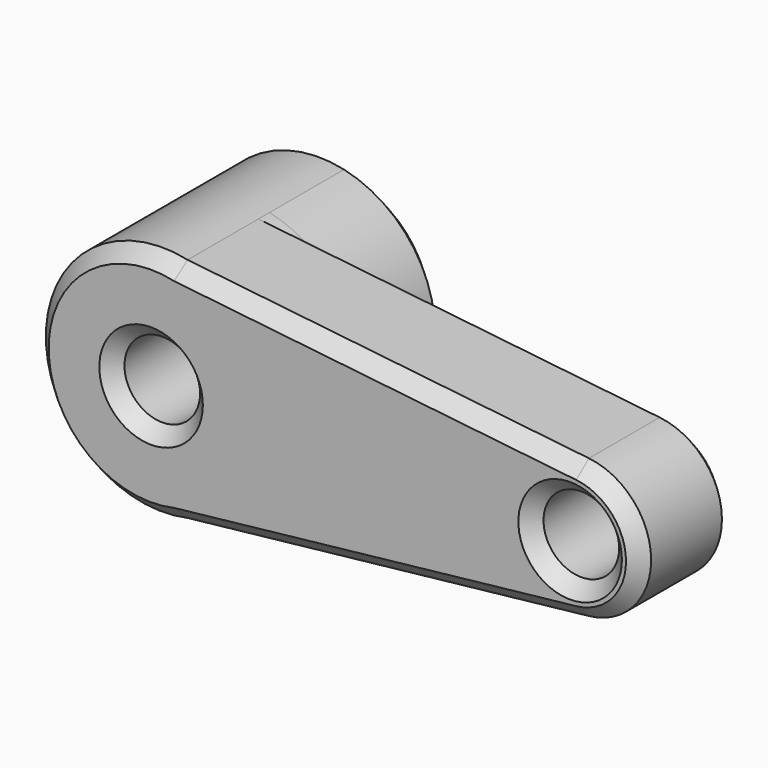
from build123d import *
from build123d import SkipClean  # not in build123d's __all__

# Parameters (mm, degrees)
F0_R         = 8.117177454
F1_DEPTH     = 25
F2_SIZE      = 3
F3_DEPTH     = 25
F4_SIZE      = 5
F5_T4_DEPTH  = 109.868464735
F5_S5_R      = 25
F5_T6_DEPTH  = 57
F5_T8_ANGLE  = 167.4336377222
F5_T12_DEPTH = 109.868464735
F5_S13_R     = 25
F5_T14_DEPTH = 57


# Not quite as in the source:
# - a fillet or chamfer that OpenCascade refuses, or shapes differently, is made with other operations: its cross-section is extruded or revolved along the edge and cut away or added


with BuildPart() as f1:
    # F0 (on Front) → F1 (new body)
    with BuildSketch(Plane.XZ):
        with BuildLine():
            ThreePointArc((5.4392563458, -24.4011165811), (19.5061709293, -15.6367930113), (25, 0))
            ThreePointArc((25, 0), (19.5061709293, 15.6367930113), (5.4392563458, 24.4011165811))
            ThreePointArc((5.4392563458, 24.4011165811), (-25, 0), (5.4392563458, -24.4011165811))
        make_face()
        Circle(F0_R, mode=Mode.SUBTRACT)
        with BuildLine():
            ThreePointArc((5.4392563458, 24.4011165811), (19.5061709293, 15.6367930113), (25, 0))
            ThreePointArc((25, 0), (19.5061709293, -15.6367930113), (5.4392563458, -24.4011165811))
            Line((5.4392563458, -24.4011165811), (91.6416380189, -14.909896868))
            ThreePointArc((91.6416380189, -14.909896868), (75, 0), (91.6416380189, 14.909896868))
            Line((91.6416380189, 14.909896868), (5.4392563458, 24.4011165811))
        make_face()
        with BuildLine():
            ThreePointArc((105, 0), (101.1719418698, 10.0093813424), (91.6416380189, 14.909896868))
            ThreePointArc((91.6416380189, 14.909896868), (75, 0), (91.6416380189, -14.909896868))
            ThreePointArc((91.6416380189, -14.909896868), (101.1719418698, -10.0093813424), (105, 0))
        make_face()
        with Locations((90, 0)):
            Circle(F0_R, mode=Mode.SUBTRACT)
    extrude(amount=F1_DEPTH)

    # F2
    f2_edges = [f1.edges().sort_by_distance(p)[0] for p in [
        (-25, -25, 0),
        (48.540447, -25, -19.655507),
        (105, -25, 0),
        (48.540447, -25, 19.655507),
        (-8.117177, -25, 0),
        (81.882823, -25, 0),
    ]]
    chamfer(f2_edges, length=F2_SIZE)

    # F0 (on Front) → F3 (join)
    with BuildSketch(Plane.XZ):
        with BuildLine():
            ThreePointArc((5.4392563458, -24.4011165811), (19.5061709293, -15.6367930113), (25, 0))
            ThreePointArc((25, 0), (19.5061709293, 15.6367930113), (5.4392563458, 24.4011165811))
            ThreePointArc((5.4392563458, 24.4011165811), (-25, 0), (5.4392563458, -24.4011165811))
        make_face()
        Circle(F0_R, mode=Mode.SUBTRACT)
    with SkipClean():  # cleaning this boolean's faces spoils the solid; the shape is the same uncleaned
        extrude(amount=-F3_DEPTH)

    # F4
    f4_edges = [f1.edges().sort_by_distance(p)[0] for p in [
        (-5.439256, 25, 24.401117),
        (-8.117177, 25, 0),
    ]]
    chamfer(f4_edges, length=F4_SIZE)

    # F5: chamfer of 3 on 1 edges, made by hand


with BuildPart() as f5_tool2:
    # F5_s3 → F5_t4 (new body)
    with BuildSketch(Plane(origin=(88.922009846, 0, -9.7906614225), x_dir=(0, 1, 0), z_dir=(-0.9939931245, 0, 0.1094425346))):
        Polygon((0, -21.8498281134), (-3, -24.8498281134), (0, -24.8498281134), align=None)
    extrude(amount=F5_T4_DEPTH)

    # F5_s5 → F5_t6 (cut, symmetric)
    with BuildSketch(Plane.XZ.offset(1.5)):
        Circle(F5_S5_R)
    extrude(amount=F5_T6_DEPTH, both=True, mode=Mode.SUBTRACT)


with BuildPart() as f1_1:
    add(f1.part, clean=False)

    # F5_t1: cut F5_tool2
    add(f5_tool2.part, mode=Mode.SUBTRACT)

    # F5_s7 → F5_t8 (revolve, cut)
    with BuildSketch(Plane(origin=(88.922009846, 0, 9.7906614225), x_dir=(0, 1, 0), z_dir=(-0.9939931245, 0, -0.1094425346))):
        Polygon((0, 21.8498281134), (-3, 24.8498281134), (0, 24.8498281134), align=None)
    revolve(axis=Axis((90, 0, 0), (0, -1, 0)), revolution_arc=F5_T8_ANGLE, mode=Mode.SUBTRACT)


with BuildPart() as f5_tool10:
    # F5_s11 → F5_t12 (new body)
    with BuildSketch(Plane(origin=(-20.2864887038, 0, -2.2336218299), x_dir=(0, 1, 0), z_dir=(0.9939931245, 0, 0.1094425346))):
        Polygon((0, -21.8498281134), (-3, -24.8498281134), (0, -24.8498281134), align=None)
    extrude(amount=F5_T12_DEPTH)

    # F5_s13 → F5_t14 (cut, symmetric)
    with BuildSketch(Plane.XZ.offset(1.5)):
        Circle(F5_S13_R)
    extrude(amount=F5_T14_DEPTH, both=True, mode=Mode.SUBTRACT)


with BuildPart() as f1_2:
    add(f1_1.part, clean=False)

    # F5_t9: cut F5_tool10
    add(f5_tool10.part, mode=Mode.SUBTRACT)


solid = f1_2.part
